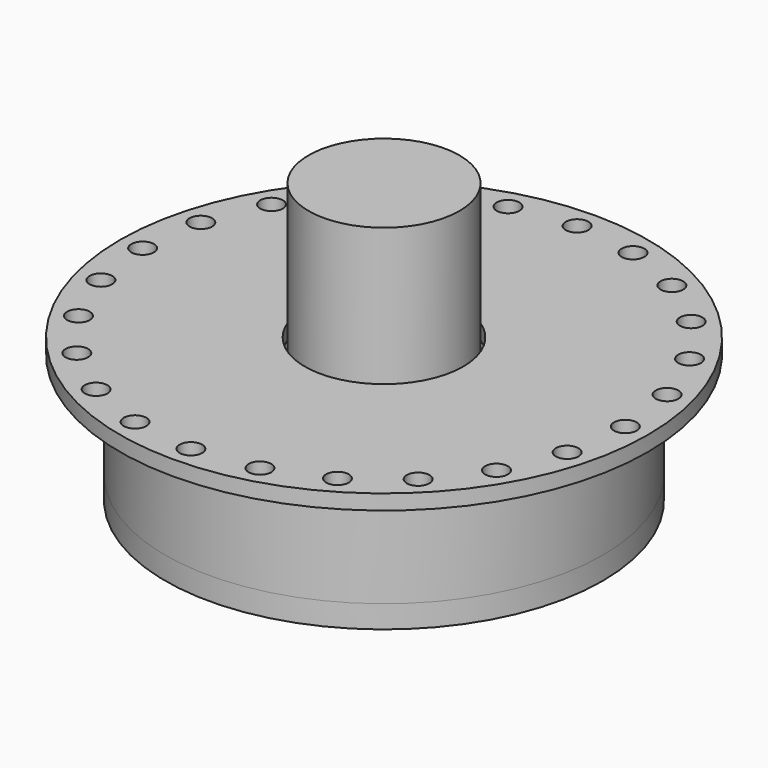
from build123d import *

# Parameters (mm, degrees)
F0_R           = 23.5
F0_R_2         = 19.5445144725
F0_R_3         = 14.0378467766
F0_R_4         = 10
F1_DEPTH       = 14
F2_DEPTH       = 2
F3_SIZE        = 2
F4_SIZE        = 1
F5_R           = 19.5445144725
F5_R_2         = 14.0378467766
F6_DEPTH       = 2
F7_R           = 35
F7_R_2         = 1.5
F7_R_3         = 10.5
F8_DEPTH       = 2
F9_R           = 29
F9_R_2         = 14.0378467766
F9_R_3         = 11
F10_DEPTH      = 13.5
F10_DEPTH_BACK = 3
F11_DEPTH      = 14
F12_DEPTH      = 20
F12_DEPTH_BACK = 25
F13_R          = 1.5
F14_DEPTH      = 37.001
F15_R          = 1.5
F16_DEPTH      = 2


with BuildPart() as f1:
    # F0 (on Top) → F1 (new body)
    with BuildSketch(Plane.XY):
        Circle(F0_R)
        Circle(F0_R_2, mode=Mode.SUBTRACT)
        Circle(F0_R_2)
        Circle(F0_R_3, mode=Mode.SUBTRACT)
        Circle(F0_R_3)
        Circle(F0_R_4, mode=Mode.SUBTRACT)
    extrude(amount=-F1_DEPTH)

    # F0 (on Top) → F2 (cut)
    with BuildSketch(Plane.XY):
        Circle(F0_R_2)
        Circle(F0_R_3, mode=Mode.SUBTRACT)
    extrude(amount=-F2_DEPTH, mode=Mode.SUBTRACT)

    # F3
    f3_edges = [f1.edges().sort_by_distance(p)[0] for p in [
        (-23.5, 0, 0),
        (-23.5, 0, -14),
    ]]
    chamfer(f3_edges, length=F3_SIZE)

    # F4
    f4_edges = [f1.edges().sort_by_distance(p)[0] for p in [
        (-10, 0, -14),
        (-10, 0, 0),
    ]]
    chamfer(f4_edges, length=F4_SIZE)

    # F5 (on face) → F6 (cut)
    with BuildSketch(Plane(origin=(0, 0, -14), x_dir=(1, 0, 0), z_dir=(0, 0, -1))):
        Circle(F5_R)
        Circle(F5_R_2, mode=Mode.SUBTRACT)
    extrude(amount=-F6_DEPTH, mode=Mode.SUBTRACT)


with BuildPart() as f8:
    # F7 (on Top) → F8 (new body)
    with BuildSketch(Plane.XY):
        Circle(F7_R)
        with Locations((-22.627416998, -22.627416998)):
            Circle(F7_R_2, mode=Mode.SUBTRACT)
        with Locations((-16, -27.7128129211)):
            Circle(F7_R_2, mode=Mode.SUBTRACT)
        with Locations((-8.2822094433, -30.9096264413)):
            Circle(F7_R_2, mode=Mode.SUBTRACT)
        with Locations((-27.7128129211, -16)):
            Circle(F7_R_2, mode=Mode.SUBTRACT)
        with Locations((-30.9096264413, -8.2822094433)):
            Circle(F7_R_2, mode=Mode.SUBTRACT)
        with Locations((0, -32)):
            Circle(F7_R_2, mode=Mode.SUBTRACT)
        with Locations((8.2822094433, -30.9096264413)):
            Circle(F7_R_2, mode=Mode.SUBTRACT)
        with Locations((16, -27.7128129211)):
            Circle(F7_R_2, mode=Mode.SUBTRACT)
        with Locations((22.627416998, -22.627416998)):
            Circle(F7_R_2, mode=Mode.SUBTRACT)
        with Locations((27.7128129211, -16)):
            Circle(F7_R_2, mode=Mode.SUBTRACT)
        with Locations((30.9096264413, -8.2822094433)):
            Circle(F7_R_2, mode=Mode.SUBTRACT)
        with Locations((-32, 0)):
            Circle(F7_R_2, mode=Mode.SUBTRACT)
        with Locations((-30.9096264413, 8.2822094433)):
            Circle(F7_R_2, mode=Mode.SUBTRACT)
        with Locations((-27.7128129211, 16)):
            Circle(F7_R_2, mode=Mode.SUBTRACT)
        with Locations((-22.627416998, 22.627416998)):
            Circle(F7_R_2, mode=Mode.SUBTRACT)
        with Locations((-16, 27.7128129211)):
            Circle(F7_R_2, mode=Mode.SUBTRACT)
        with Locations((-8.2822094433, 30.9096264413)):
            Circle(F7_R_2, mode=Mode.SUBTRACT)
        Circle(F7_R_3, mode=Mode.SUBTRACT)
        with Locations((32, 0)):
            Circle(F7_R_2, mode=Mode.SUBTRACT)
        with Locations((30.9096264413, 8.2822094433)):
            Circle(F7_R_2, mode=Mode.SUBTRACT)
        with Locations((27.7128129211, 16)):
            Circle(F7_R_2, mode=Mode.SUBTRACT)
        with Locations((0, 32)):
            Circle(F7_R_2, mode=Mode.SUBTRACT)
        with Locations((8.2822094433, 30.9096264413)):
            Circle(F7_R_2, mode=Mode.SUBTRACT)
        with Locations((16, 27.7128129211)):
            Circle(F7_R_2, mode=Mode.SUBTRACT)
        with Locations((22.627416998, 22.627416998)):
            Circle(F7_R_2, mode=Mode.SUBTRACT)
    extrude(amount=F8_DEPTH)


with BuildPart() as f10:
    # F9 (on face) → F10 (new body, two sides)
    with BuildSketch(Plane(origin=(0, 0, -14), x_dir=(1, 0, 0), z_dir=(0, 0, -1))) as f10_sk:
        Circle(F9_R)
        Circle(F9_R_2, mode=Mode.SUBTRACT)
        Circle(F9_R_2)
        Circle(F9_R_3, mode=Mode.SUBTRACT)
    extrude(amount=-F10_DEPTH)
    extrude(f10_sk.sketch, amount=F10_DEPTH_BACK)

    # F0 (on Top) → F11 (cut, through all)
    with BuildSketch(Plane.XY):
        Circle(F0_R)
        Circle(F0_R_2, mode=Mode.SUBTRACT)
        Circle(F0_R_2)
        Circle(F0_R_3, mode=Mode.SUBTRACT)
        Circle(F0_R_3)
        Circle(F0_R_4, mode=Mode.SUBTRACT)
    extrude(amount=-F11_DEPTH, mode=Mode.SUBTRACT)

    # F13 (on face) → F14 (cut, through all)
    with BuildSketch(Plane(origin=(0, 0, -17), x_dir=(1, 0, 0), z_dir=(0, 0, -1))):
        with Locations((0, 25.5)):
            Circle(F13_R)
        with Locations((-22.0836477965, 12.75)):
            Circle(F13_R)
        with Locations((-22.0836477965, -12.75)):
            Circle(F13_R)
        with Locations((0, -25.5)):
            Circle(F13_R)
        with Locations((22.0836477965, 12.75)):
            Circle(F13_R)
        with Locations((22.0836477965, -12.75)):
            Circle(F13_R)
    extrude(amount=-F14_DEPTH, mode=Mode.SUBTRACT)

    # F15 (on face) → F16 (cut)
    with BuildSketch(Plane(origin=(0, 0, -17), x_dir=(1, 0, 0), z_dir=(0, 0, -1))):
        Polygon((-1.5, 22.9019237886), (1.5, 22.9019237886), (3, 25.5), (1.5, 28.0980762114), (-1.5, 28.0980762114), (-3, 25.5), align=None)
        with Locations((0, 25.5)):
            Circle(F15_R, mode=Mode.SUBTRACT)
        Polygon((-25.0836477965, 12.75), (-23.5836477965, 10.1519237886), (-20.5836477965, 10.1519237886), (-19.0836477965, 12.75), (-20.5836477965, 15.3480762114), (-23.5836477965, 15.3480762114), align=None)
        with Locations((-22.0836477965, 12.75)):
            Circle(F15_R, mode=Mode.SUBTRACT)
        Polygon((-23.5836477965, -15.3480762114), (-20.5836477965, -15.3480762114), (-19.0836477965, -12.75), (-20.5836477965, -10.1519237886), (-23.5836477965, -10.1519237886), (-25.0836477965, -12.75), align=None)
        with Locations((-22.0836477965, -12.75)):
            Circle(F15_R, mode=Mode.SUBTRACT)
        Polygon((23.5836477965, 15.3480762114), (20.5836477965, 15.3480762114), (19.0836477965, 12.75), (20.5836477965, 10.1519237886), (23.5836477965, 10.1519237886), (25.0836477965, 12.75), align=None)
        with Locations((22.0836477965, 12.75)):
            Circle(F15_R, mode=Mode.SUBTRACT)
        Polygon((25.0836477965, -12.75), (23.5836477965, -10.1519237886), (20.5836477965, -10.1519237886), (19.0836477965, -12.75), (20.5836477965, -15.3480762114), (23.5836477965, -15.3480762114), align=None)
        with Locations((22.0836477965, -12.75)):
            Circle(F15_R, mode=Mode.SUBTRACT)
        Polygon((1.5, -28.0980762114), (3, -25.5), (1.5, -22.9019237886), (-1.5, -22.9019237886), (-3, -25.5), (-1.5, -28.0980762114), align=None)
        with Locations((0, -25.5)):
            Circle(F15_R, mode=Mode.SUBTRACT)
    extrude(amount=-F16_DEPTH, mode=Mode.SUBTRACT)


with BuildPart() as f12:
    # F0 (on Top) → F12 (new body, two sides)
    with BuildSketch(Plane.XY) as f12_sk:
        Circle(F0_R_4)
    extrude(amount=F12_DEPTH)
    extrude(f12_sk.sketch, amount=-F12_DEPTH_BACK)


solid = Compound([f1.part, f8.part, f10.part, f12.part])
